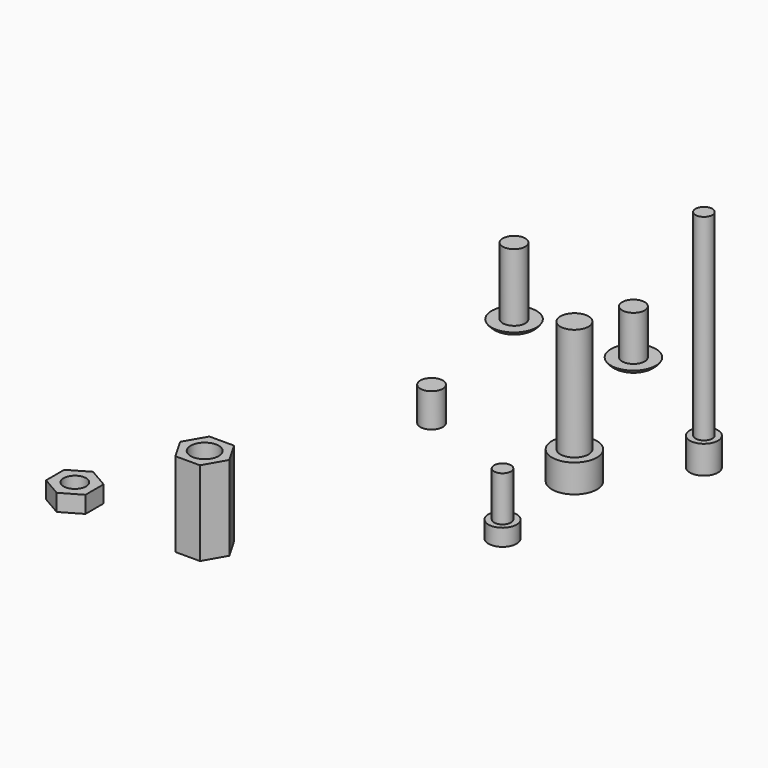
from build123d import *

# Parameters (mm, degrees)
F0_R      = 2
F1_DEPTH  = 6
F0_R_2    = 1.5
F2_DEPTH  = 8
F0_R_3    = 2.5
F3_DEPTH  = 3
F4_DEPTH  = 20
F0_R_4    = 4
F5_DEPTH  = 5
F6_DEPTH  = 3
F7_DEPTH  = 8
F8_DEPTH  = 1
F10_DEPTH = 35
F11_DEPTH = 3
F12_DEPTH = 12
F13_DEPTH = 15


# Not quite as in the source:
# - a fillet or chamfer that OpenCascade refuses, or shapes differently, is made with other operations: its cross-section is extruded or revolved along the edge and cut away or added


with BuildPart() as f1:
    # F0 (on Top) → F1 (new body)
    with BuildSketch(Plane.XY):
        with Locations((-0.1684613526, 0.2074986696)):
            Circle(F0_R)
        Polygon((-1.3072340101, 0.7229565578), (-0.2914480557, 1.4514336643), (0.8473246019, 0.9359757761), (0.970311305, -0.3079592185), (-0.0454746495, -1.036436325), (-1.1842473071, -0.5209784369), align=None, mode=Mode.SUBTRACT)
        Polygon((0.8473246019, 0.9359757761), (-0.2914480557, 1.4514336643), (-1.3072340101, 0.7229565578), (-1.1842473071, -0.5209784369), (-0.0454746495, -1.036436325), (0.970311305, -0.3079592185), align=None)
    extrude(amount=F1_DEPTH)

    # F0 (on Top) → F6 (cut)
    with BuildSketch(Plane.XY):
        Polygon((0.8473246019, 0.9359757761), (-0.2914480557, 1.4514336643), (-1.3072340101, 0.7229565578), (-1.1842473071, -0.5209784369), (-0.0454746495, -1.036436325), (0.970311305, -0.3079592185), align=None)
    extrude(amount=F6_DEPTH, mode=Mode.SUBTRACT)


with BuildPart() as f2:
    # F0 (on Top) → F2 (new body)
    with BuildSketch(Plane.XY):
        with Locations((25.6595015526, -16.3031816483)):
            Circle(F0_R_2)
        Polygon((24.520728895, -15.7877237601), (25.5365148495, -15.0592466536), (26.6752875071, -15.5747045418), (26.7982742101, -16.8186395364), (25.7824882557, -17.5471166429), (24.6437155981, -17.0316587548), align=None, mode=Mode.SUBTRACT)
        Polygon((26.6752875071, -15.5747045418), (25.5365148495, -15.0592466536), (24.520728895, -15.7877237601), (24.6437155981, -17.0316587548), (25.7824882557, -17.5471166429), (26.7982742101, -16.8186395364), align=None)
    extrude(amount=F2_DEPTH)

    # F0 (on Top) → F3 (join)
    with BuildSketch(Plane.XY):
        with Locations((25.6595015526, -16.3031816483)):
            Circle(F0_R_3)
        with Locations((25.6595015526, -16.3031816483)):
            Circle(F0_R_2, mode=Mode.SUBTRACT)
        with Locations((25.6595015526, -16.3031816483)):
            Circle(F0_R_2)
        Polygon((24.520728895, -15.7877237601), (25.5365148495, -15.0592466536), (26.6752875071, -15.5747045418), (26.7982742101, -16.8186395364), (25.7824882557, -17.5471166429), (24.6437155981, -17.0316587548), align=None, mode=Mode.SUBTRACT)
    extrude(amount=-F3_DEPTH)


with BuildPart() as f4:
    # F0 (on Top) → F4 (new body)
    with BuildSketch(Plane.XY):
        with Locations((20.266674459, 6.419762969)):
            Circle(F0_R_3)
        Polygon((19.1841427043, 7.044762969), (20.266674459, 7.669762969), (21.3492062137, 7.044762969), (21.3492062137, 5.794762969), (20.266674459, 5.169762969), (19.1841427043, 5.794762969), align=None, mode=Mode.SUBTRACT)
        Polygon((21.3492062137, 7.044762969), (20.266674459, 7.669762969), (19.1841427043, 7.044762969), (19.1841427043, 5.794762969), (20.266674459, 5.169762969), (21.3492062137, 5.794762969), align=None)
    extrude(amount=F4_DEPTH)

    # F0 (on Top) → F5 (join)
    with BuildSketch(Plane.XY):
        with Locations((20.266674459, 6.419762969)):
            Circle(F0_R_4)
        with Locations((20.266674459, 6.419762969)):
            Circle(F0_R_3, mode=Mode.SUBTRACT)
        with Locations((20.266674459, 6.419762969)):
            Circle(F0_R_3)
        Polygon((19.1841427043, 7.044762969), (20.266674459, 7.669762969), (21.3492062137, 7.044762969), (21.3492062137, 5.794762969), (20.266674459, 5.169762969), (19.1841427043, 5.794762969), align=None, mode=Mode.SUBTRACT)
    extrude(amount=-F5_DEPTH)


with BuildPart() as f5:
    # F0 (on Top) → F5, piece 2 (new body)
    with BuildSketch(Plane.XY):
        with Locations((31.7245647311, 20.8836849779)):
            Circle(F0_R_3)
        with Locations((31.7245647311, 20.8836849779)):
            Circle(F0_R_2, mode=Mode.SUBTRACT)
        with Locations((31.7245647311, 20.8836849779)):
            Circle(F0_R_2)
        Polygon((30.6420329764, 21.5086849779), (31.7245647311, 22.1336849779), (32.8070964859, 21.5086849779), (32.8070964859, 20.2586849779), (31.7245647311, 19.6336849779), (30.6420329764, 20.2586849779), align=None, mode=Mode.SUBTRACT)
    extrude(amount=-F5_DEPTH)

    # F0 (on Top) → F10 (join)
    with BuildSketch(Plane.XY):
        with Locations((31.7245647311, 20.8836849779)):
            Circle(F0_R_2)
        Polygon((30.6420329764, 21.5086849779), (31.7245647311, 22.1336849779), (32.8070964859, 21.5086849779), (32.8070964859, 20.2586849779), (31.7245647311, 19.6336849779), (30.6420329764, 20.2586849779), align=None, mode=Mode.SUBTRACT)
        Polygon((32.8070964859, 21.5086849779), (31.7245647311, 22.1336849779), (30.6420329764, 21.5086849779), (30.6420329764, 20.2586849779), (31.7245647311, 19.6336849779), (32.8070964859, 20.2586849779), align=None)
    extrude(amount=F10_DEPTH)


with BuildPart() as f7:
    # F0 (on Top) → F7 (new body)
    with BuildSketch(Plane.XY):
        with Locations((9.3955630437, 33.1254936755)):
            Circle(F0_R)
        Polygon((8.3130312889, 33.7504936755), (9.3955630437, 34.3754936755), (10.4780947984, 33.7504936755), (10.4780947984, 32.5004936755), (9.3955630437, 31.8754936755), (8.3130312889, 32.5004936755), align=None, mode=Mode.SUBTRACT)
        Polygon((10.4780947984, 33.7504936755), (9.3955630437, 34.3754936755), (8.3130312889, 33.7504936755), (8.3130312889, 32.5004936755), (9.3955630437, 31.8754936755), (10.4780947984, 32.5004936755), align=None)
    extrude(amount=F7_DEPTH)

    # F0 (on Top) → F8 (join)
    with BuildSketch(Plane.XY):
        with Locations((9.3955630437, 33.1254936755)):
            Circle(F0_R_4)
        with Locations((9.3955630437, 33.1254936755)):
            Circle(F0_R, mode=Mode.SUBTRACT)
        with Locations((9.3955630437, 33.1254936755)):
            Circle(F0_R)
        Polygon((8.3130312889, 33.7504936755), (9.3955630437, 34.3754936755), (10.4780947984, 33.7504936755), (10.4780947984, 32.5004936755), (9.3955630437, 31.8754936755), (8.3130312889, 32.5004936755), align=None, mode=Mode.SUBTRACT)
    extrude(amount=-F8_DEPTH)

    # F9: fillet of radius 2 on 1 edges, made by hand

    # F9_s1 → F9_t2 (revolve, cut)
    with BuildSketch(Plane.XZ.offset(-33.1254936755)):
        with BuildLine():
            ThreePointArc((13.3955630437, 0), (12.6635122361, -0.7320508076), (11.6635122361, -1))
            Line((11.6635122361, -1), (13.3955630437, -1))
            Line((13.3955630437, -1), (13.3955630437, 0))
        make_face()
    revolve(axis=Axis((9.3955630437, 33.1254936755, -1), (0, 0, 1)), mode=Mode.SUBTRACT)


with BuildPart() as f8:
    # F0 (on Top) → F8, piece 2 (new body)
    with BuildSketch(Plane.XY):
        with Locations((-10.7167446986, 31.7254327238)):
            Circle(F0_R_4)
        with Locations((-10.7167446986, 31.7254327238)):
            Circle(F0_R, mode=Mode.SUBTRACT)
        with Locations((-10.7167446986, 31.7254327238)):
            Circle(F0_R)
        Polygon((-11.7992764533, 32.3504327238), (-10.7167446986, 32.9754327238), (-9.6342129439, 32.3504327238), (-9.6342129439, 31.1004327238), (-10.7167446986, 30.4754327238), (-11.7992764533, 31.1004327238), align=None, mode=Mode.SUBTRACT)
    extrude(amount=-F8_DEPTH)

    # F9#2: fillet of radius 2 on 1 edges, made by hand

    # F9_2_s1 → F9_2_t2 (revolve, cut)
    with BuildSketch(Plane.XZ.offset(-31.7254327238)):
        with BuildLine():
            ThreePointArc((-6.7167446986, 0), (-7.4487955062, -0.7320508076), (-8.4487955062, -1))
            Line((-8.4487955062, -1), (-6.7167446986, -1))
            Line((-6.7167446986, -1), (-6.7167446986, 0))
        make_face()
    revolve(axis=Axis((-10.7167446986, 31.7254327238, -1), (0, 0, 1)), mode=Mode.SUBTRACT)

    # F0 (on Top) → F12 (join)
    with BuildSketch(Plane.XY):
        with Locations((-10.7167446986, 31.7254327238)):
            Circle(F0_R)
        Polygon((-11.7992764533, 32.3504327238), (-10.7167446986, 32.9754327238), (-9.6342129439, 32.3504327238), (-9.6342129439, 31.1004327238), (-10.7167446986, 30.4754327238), (-11.7992764533, 31.1004327238), align=None, mode=Mode.SUBTRACT)
        Polygon((-9.6342129439, 32.3504327238), (-10.7167446986, 32.9754327238), (-11.7992764533, 32.3504327238), (-11.7992764533, 31.1004327238), (-10.7167446986, 30.4754327238), (-9.6342129439, 31.1004327238), align=None)
    extrude(amount=F12_DEPTH)


with BuildPart() as f11:
    # F0 (on Top) → F11 (new body)
    with BuildSketch(Plane.XY):
        Polygon((-20.59273386, -51.1970724528), (-20.59273386, -47.1556205685), (-24.09273386, -45.1348946263), (-27.59273386, -47.1556205685), (-27.59273386, -51.1970724528), (-24.09273386, -53.217798395), align=None)
        with Locations((-24.09273386, -49.1763465106)):
            Circle(F0_R, mode=Mode.SUBTRACT)
    extrude(amount=F11_DEPTH)


with BuildPart() as f13:
    # F0 (on Top) → F13 (new body)
    with BuildSketch(Plane.XY):
        Polygon((0.6715684338, -52.3293341259), (2.8590684338, -48.5404729843), (0.6715684338, -44.7516118428), (-3.7034315662, -44.7516118428), (-5.8909315662, -48.5404729843), (-3.7034315662, -52.3293341259), align=None)
        with Locations((-1.5159315662, -48.5404729843)):
            Circle(F0_R_3, mode=Mode.SUBTRACT)
    extrude(amount=F13_DEPTH)


solid = Compound([f1.part, f2.part, f4.part, f5.part, f7.part, f8.part, f11.part, f13.part])
